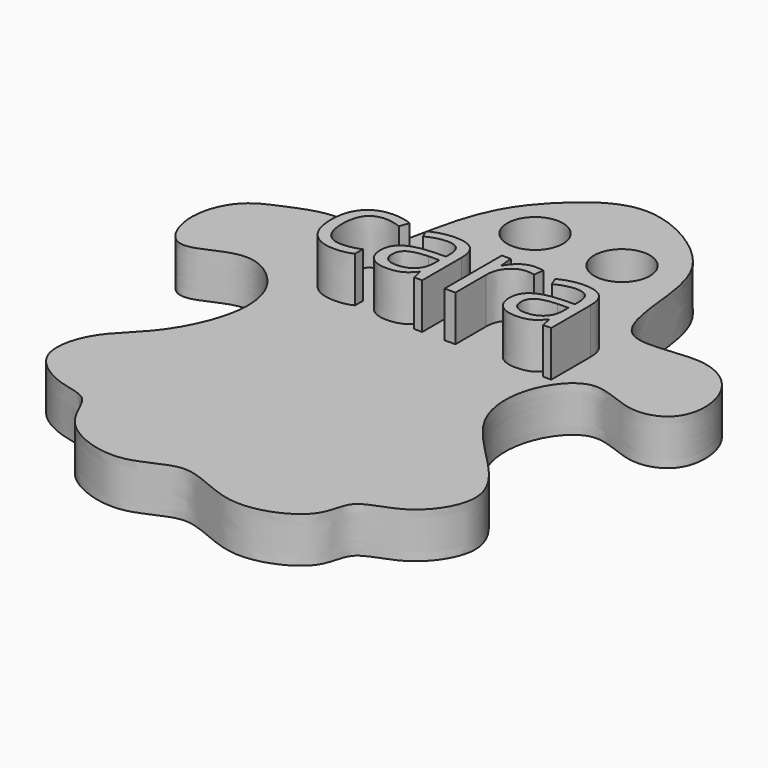
from build123d import *

# Parameters (mm, degrees)
F0_R         = 2.4501322643
F1_DEPTH     = 4
F2_TEXT_SIZE = 11.7581492911
F3_DEPTH     = 4


# Not quite as in the source:
# - Text() gives the source's letters only with a copy of the font that has no kerning and outlines rounded to 1/6400 em; it was checked with that copy


with BuildPart() as f1:
    # F0 (on Top) → F1 (new body)
    with BuildSketch(Plane.XY):
        with BuildLine():
            add(Edge.make_bspline(
                [(-56.233111769, 62.677256763), (-56.950869265, 61.3006956125), (-57.9068343584, 58.235500039), (-58.6257091192, 52.692580614), (-63.6882787465, 55.8030426481), (-67.980424745, 53.9118120871), (-70.9481153276, 52.6995380188), (-72.5715487105, 48.6345192061), (-70.5764037553, 44.0634422633), (-66.8429647206, 46.4237907066), (-64.0345652573, 46.6266985999), (-60.9131161908, 43.9391520364), (-60.3528142584, 39.4024630362), (-62.9422744978, 33.8619952762), (-66.5594126095, 31.2019958284), (-67.7580174314, 26.1455004683), (-63.6151530841, 23.6275024833), (-60.4963197631, 23.5153514202), (-59.7648836543, 19.1467817922), (-53.1766725617, 16.6685019481), (-48.9133259254, 20.5112305067), (-43.5269641603, 16.2498358578), (-37.0032883521, 19.1361019847), (-37.2660976885, 22.9198156593), (-32.7717937531, 23.4405010413), (-29.2901286564, 28.8099087368), (-34.0399123616, 33.7457065681), (-38.2845910818, 37.9422106241), (-38.3414623821, 43.4891878633), (-34.9438691638, 47.5312568704), (-30.7760418018, 44.6706374535), (-26.6552103091, 46.043556443), (-26.5709255482, 51.20630811), (-30.8316700961, 54.8824386103), (-38.799670189, 52.0367863827), (-38.9220406782, 60.97018514), (-40.6877273736, 65.9860607805), (-48.4289828196, 70.4265248926), (-53.7141607957, 66.2848556754), (-55.562314921, 63.9637537844), (-56.233111769, 62.677256763)],
                knots=[0, 0, 0, 0, 0.0275920863, 0.0523103128, 0.0777917567, 0.1040501151, 0.1255769621, 0.1503067905, 0.17396023, 0.1968621844, 0.2171290895, 0.2404790783, 0.2660364815, 0.2957645316, 0.3219072993, 0.3472321528, 0.3724081663, 0.3925696697, 0.4161166705, 0.4462633656, 0.47299599, 0.5027750047, 0.5326589244, 0.5533462399, 0.5772999375, 0.6051474992, 0.6353880103, 0.6654512852, 0.6931595078, 0.7180834295, 0.7434920972, 0.7663562533, 0.7916283631, 0.8188938579, 0.8495777207, 0.8814064993, 0.9106165104, 0.94440831, 0.9742131784, 1, 1, 1, 1], degree=3))
        make_face()
        with Locations((-52.0066991448, 61.5473277867)):
            Circle(F0_R, mode=Mode.SUBTRACT)
        with Locations((-44.3637161083, 61.5473277867)):
            Circle(F0_R, mode=Mode.SUBTRACT)
    extrude(amount=F1_DEPTH)

    # F2 (on face) → F3 (join)
    with BuildSketch(Plane.XY.offset(4)):
        with Locations((-60.0919794865, 45.2749564228)):
            Text('cara', F2_TEXT_SIZE, font='Open Sans', text_align=(TextAlign.LEFT, TextAlign.BOTTOM))
    extrude(amount=F3_DEPTH)


solid = f1.part
